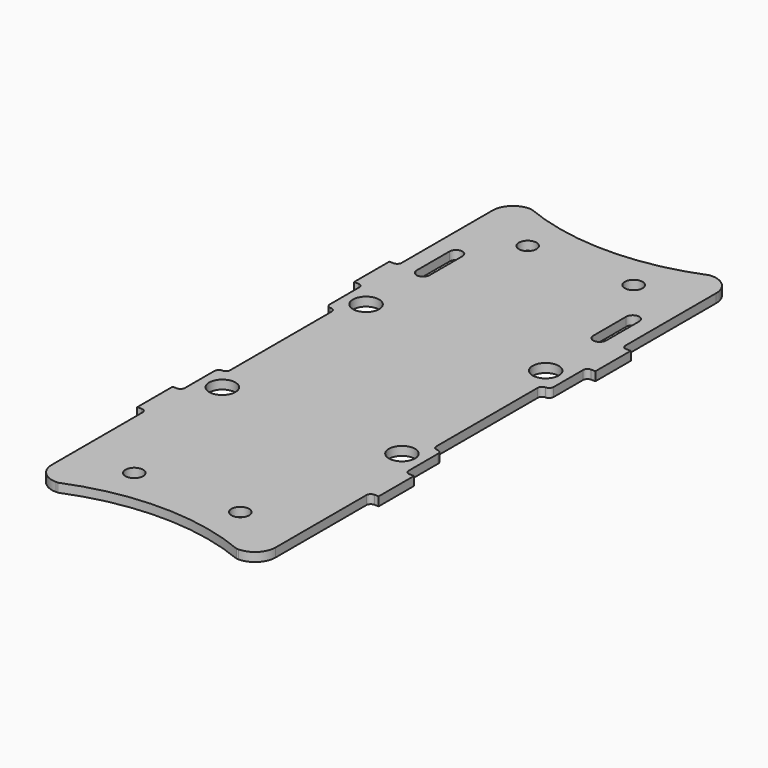
from build123d import *

# Parameters (mm, degrees)
F0_R     = 1.5
F0_R_2   = 2.225
F1_DEPTH = 1.5


# Not quite as in the source:
# - ends of sketch curves that miss each other by under 0.0002 mm in the source are joined


with BuildPart() as f1:
    # F0 (on Top) → F1 (new body)
    with BuildSketch(Plane.XY):
        with BuildLine():
            ThreePointArc((19.75, -19.25), (19.2196699141, -19.0303300859), (19, -18.5))
            Line((19, -18.5), (19, -12.25))
            ThreePointArc((19, -12.25), (18.7803300859, -11.7196699141), (18.25, -11.5))
            ThreePointArc((18.25, -11.5), (17.7196699141, -11.2803300859), (17.5, -10.75))
            Line((17.5, -10.75), (17.5, 10.75))
            ThreePointArc((17.5, 10.75), (17.7196699141, 11.2803300859), (18.25, 11.5))
            ThreePointArc((18.25, 11.5), (18.7803300859, 11.7196699141), (19, 12.25))
            Line((19, 12.25), (19, 18.5))
            ThreePointArc((19, 18.5), (19.2196699141, 19.0303300859), (19.75, 19.25))
            Line((19.75, 19.25), (20.5, 19.25))
            Line((20.5, 19.25), (20.5, 26.75))
            Line((20.5, 26.75), (19.75, 26.75))
            ThreePointArc((19.75, 26.75), (19.2196699141, 26.9696699141), (19, 27.5))
            Line((19, 27.5), (19, 46.75))
            ThreePointArc((19, 46.75), (17.9748737342, 49.2248737342), (15.5, 50.25))
            Line((15.5, 50.25), (15.167259, 50.25))
            ThreePointArc((15.167259, 50.25), (0, 47.25), (-15.1672590116, 50.2499999718))
            Line((-15.1672590116, 50.2499999718), (-15.5, 50.25))
            ThreePointArc((-15.5, 50.25), (-17.9748737342, 49.2248737342), (-19, 46.75))
            Line((-19, 46.75), (-19, 27.5))
            ThreePointArc((-19, 27.5), (-19.2196699141, 26.9696699141), (-19.75, 26.75))
            Line((-19.75, 26.75), (-20.5, 26.75))
            Line((-20.5, 26.75), (-20.5, 19.25))
            Line((-20.5, 19.25), (-19.75, 19.25))
            ThreePointArc((-19.75, 19.25), (-19.2196699141, 19.0303300859), (-19, 18.5))
            Line((-19, 18.5), (-19, 12.25))
            ThreePointArc((-19, 12.25), (-18.7803300859, 11.7196699141), (-18.25, 11.5))
            ThreePointArc((-18.25, 11.5), (-17.7196699141, 11.2803300859), (-17.5, 10.75))
            Line((-17.5, 10.75), (-17.5, -10.75))
            ThreePointArc((-17.5, -10.75), (-17.7196699141, -11.2803300859), (-18.25, -11.5))
            ThreePointArc((-18.25, -11.5), (-18.7803300859, -11.7196699141), (-19, -12.25))
            Line((-19, -12.25), (-19, -18.5))
            ThreePointArc((-19, -18.5), (-19.2196699141, -19.0303300859), (-19.75, -19.25))
            Line((-19.75, -19.25), (-20.5, -19.25))
            Line((-20.5, -19.25), (-20.5, -26.75))
            Line((-20.5, -26.75), (-19.75, -26.75))
            ThreePointArc((-19.75, -26.75), (-19.2196699141, -26.9696699141), (-19, -27.5))
            Line((-19, -27.5), (-19, -46.75))
            ThreePointArc((-19, -46.75), (-17.9748737342, -49.2248737342), (-15.5, -50.25))
            Line((-15.5, -50.25), (-15.167259, -50.25))
            ThreePointArc((-15.167259, -50.25), (0, -47.249999), (15.1672593636, -50.2499991168))
            Line((15.1672593636, -50.2499991168), (15.5, -50.25))
            ThreePointArc((15.5, -50.25), (17.9748737342, -49.2248737342), (19, -46.75))
            Line((19, -46.75), (19, -27.5))
            ThreePointArc((19, -27.5), (19.2196699141, -26.9696699141), (19.75, -26.75))
            Line((19.75, -26.75), (20.5, -26.75))
            Line((20.5, -26.75), (20.5, -19.25))
            Line((20.5, -19.25), (19.75, -19.25))
        make_face()
        with Locations((-9, -41.75)):
            Circle(F0_R, mode=Mode.SUBTRACT)
        with Locations((-15.25, -15.25)):
            Circle(F0_R_2, mode=Mode.SUBTRACT)
        with Locations((9, -41.75)):
            Circle(F0_R, mode=Mode.SUBTRACT)
        with Locations((15.25, -15.25)):
            Circle(F0_R_2, mode=Mode.SUBTRACT)
        with Locations((-15.25, 15.25)):
            Circle(F0_R_2, mode=Mode.SUBTRACT)
        with BuildLine():
            ThreePointArc((-16.1, 34.033918), (-15, 35.133918), (-13.9, 34.033918))
            Line((-13.9, 34.033918), (-13.9, 27.033918))
            ThreePointArc((-13.9, 27.033918), (-15, 25.933918), (-16.1, 27.033918))
            Line((-16.1, 27.033918), (-16.1, 34.033918))
        make_face(mode=Mode.SUBTRACT)
        with Locations((-9, 41.75)):
            Circle(F0_R, mode=Mode.SUBTRACT)
        with Locations((15.25, 15.25)):
            Circle(F0_R_2, mode=Mode.SUBTRACT)
        with Locations((9, 41.75)):
            Circle(F0_R, mode=Mode.SUBTRACT)
        with BuildLine():
            ThreePointArc((13.9, 34.033918), (15, 35.133918), (16.1, 34.033918))
            Line((16.1, 34.033918), (16.1, 27.033918))
            ThreePointArc((16.1, 27.033918), (15, 25.933918), (13.9, 27.033918))
            Line((13.9, 27.033918), (13.9, 34.033918))
        make_face(mode=Mode.SUBTRACT)
    extrude(amount=F1_DEPTH)


solid = f1.part
